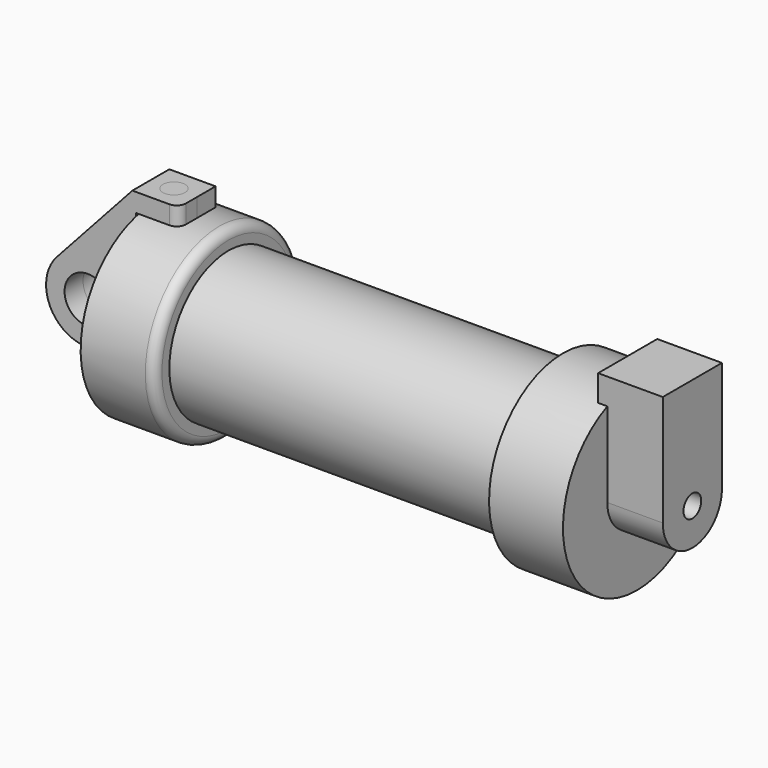
from build123d import *

# Parameters (mm, degrees)
F0_W     = 5.842
F0_H     = 12.7
F0_R     = 3.175
F2_DEPTH = 3.175
F4_DEPTH = 1.27
F3_R     = 1.524
F5_DEPTH = 7.62
F6_R     = 1.524
F8_DEPTH = 17.78
F10_R    = 1.27
F11_R    = 1.27


# Not quite as in the source:
# - the program builds the solid bodies; features that only make, move or delete a surface that nothing else refers to are left out


with BuildPart() as f1:
    # F0 (on Front) → F1 (revolve)
    with BuildSketch(Plane.XZ):
        with Locations((2.921, 6.35)):
            Rectangle(F0_W, F0_H)
        Polygon((5.842, 12.7), (5.842, 0), (66.294, 0), (66.294, 12.7), (56.134, 12.7), (56.134, 10.16), (10.16, 10.16), (10.16, 12.7), align=None)
    revolve(axis=Axis((33.147, 0, 0), (-1, 0, 0)))

    # F3 (on face) → F4 (join)
    with BuildSketch(Plane.YZ.offset(66.294)):
        with BuildLine():
            ThreePointArc((-5.08, 11.6397422652), (0, 12.7), (5.08, 11.6397422652))
            Line((5.08, 11.6397422652), (5.08, 15.24))
            Line((5.08, 15.24), (-5.08, 15.24))
            Line((-5.08, 15.24), (-5.08, 11.6397422652))
        make_face()
    extrude(amount=-F4_DEPTH)

    # F3 (on face) → F5 (join)
    with BuildSketch(Plane.YZ.offset(66.294)):
        with BuildLine():
            ThreePointArc((-5.08, 0), (0, -5.08), (5.08, 0))
            ThreePointArc((5.08, 0), (0, 5.08), (-5.08, 0))
        make_face()
        Circle(F3_R, mode=Mode.SUBTRACT)
        with BuildLine():
            ThreePointArc((-5.08, 0), (0, 5.08), (5.08, 0))
            Line((5.08, 0), (5.08, 15.24))
            Line((5.08, 15.24), (-5.08, 15.24))
            Line((-5.08, 15.24), (-5.08, 0))
        make_face()
    extrude(amount=F5_DEPTH)

    # F10
    f10_edges = [f1.edges().sort_by_distance(p)[0] for p in [
        (10.16, 0, -12.7),
    ]]
    fillet(f10_edges, radius=F10_R)


with BuildPart() as f2:
    # F0 (on Front) → F2 (new body, symmetric)
    with BuildSketch(Plane.XZ):
        with BuildLine():
            Line((-0.9398, 0), (0, 0))
            Line((0, 0), (0, 12.7))
            Line((0, 12.7), (5.842, 12.7))
            Line((5.842, 12.7), (5.842, 15.24))
            Line((5.842, 15.24), (-0.508, 15.24))
            Line((-0.508, 15.24), (-10.8806298187, 3.8475430269))
            ThreePointArc((-10.8806298187, 3.8475430269), (-4.5919612295, 5.3297205562), (-0.9398, 0))
        make_face()
        with BuildLine():
            ThreePointArc((-8.1826630726, -5.5069827884), (-3.1957909266, -4.5493385486), (-0.9398, 0))
            ThreePointArc((-0.9398, 0), (-4.5919612295, 5.3297205562), (-10.8806298187, 3.8475430269))
            ThreePointArc((-10.8806298187, 3.8475430269), (-12.1459778134, -1.5837270034), (-8.1826630726, -5.5069827884))
        make_face()
        with Locations((-6.6548, 0)):
            Circle(F0_R, mode=Mode.SUBTRACT)
    extrude(amount=F2_DEPTH, both=True)

    # F11
    f11_edges = [f2.edges().sort_by_distance(p)[0] for p in [
        (5.842, -3.175, 13.97),
    ]]
    fillet(f11_edges, radius=F11_R)


with BuildPart() as f8:
    # F6 (on face) → F8 (new body)
    with BuildSketch(Plane.XY.offset(15.24)):
        with Locations((2.667, 0)):
            Circle(F6_R)
    extrude(amount=-F8_DEPTH)


solid = Compound([f1.part, f2.part, f8.part])
